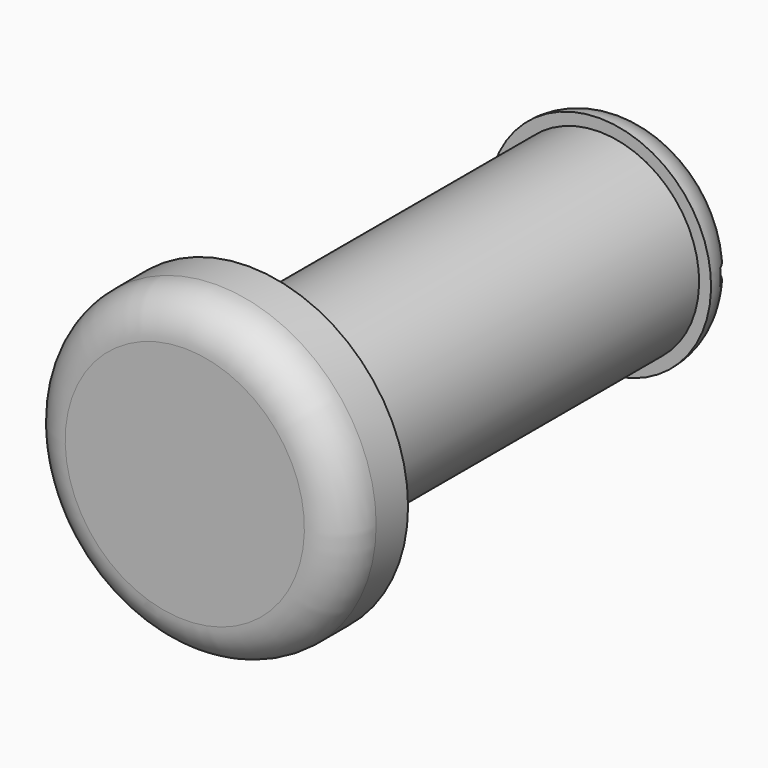
from build123d import *

# Parameters (mm, degrees)
F2_R     = 0.5
F3_R     = 0.49999
F4_W     = 3
F4_H     = 0.1
F5_DEPTH = 0.3


# Not quite as in the source:
# - a fillet or chamfer is up to 0.001 mm smaller than in the source, because OpenCascade refuses the exact size


with BuildPart() as f1:
    # F0 (on Right) → F1 (revolve)
    with BuildSketch(Plane.YZ):
        Polygon((-3.5, 0), (-2.5, 0), (3, 0), (3.5, 0), (3.5, 1.4), (3, 1.4), (3, 1.25), (-2.5, 1.25), (-2.5, 2), (-3.5, 2), align=None)
    revolve(axis=Axis((0, 0.25, 0), (0, -1, 0)))

    # F2
    f2_edges = [f1.edges().sort_by_distance(p)[0] for p in [
        (0, -3.5, -2),
    ]]
    fillet(f2_edges, radius=F2_R)

    # F3 (radius 0.5 in the source; OpenCascade refuses exactly that, so slightly less here)
    f3_edges = [f1.edges().sort_by_distance(p)[0] for p in [
        (0, 3.5, -1.4),
    ]]
    fillet(f3_edges, radius=F3_R)

    # F4 (on face) → F5 (cut)
    with BuildSketch(Plane(origin=(0, 3.5, 0), x_dir=(-1, 0, 0), z_dir=(0, 1, 0))):
        with Locations((0, 0.05)):
            Rectangle(F4_W, F4_H)
        with Locations((0, -0.05)):
            Rectangle(F4_W, F4_H)
    extrude(amount=-F5_DEPTH, mode=Mode.SUBTRACT)


solid = f1.part
